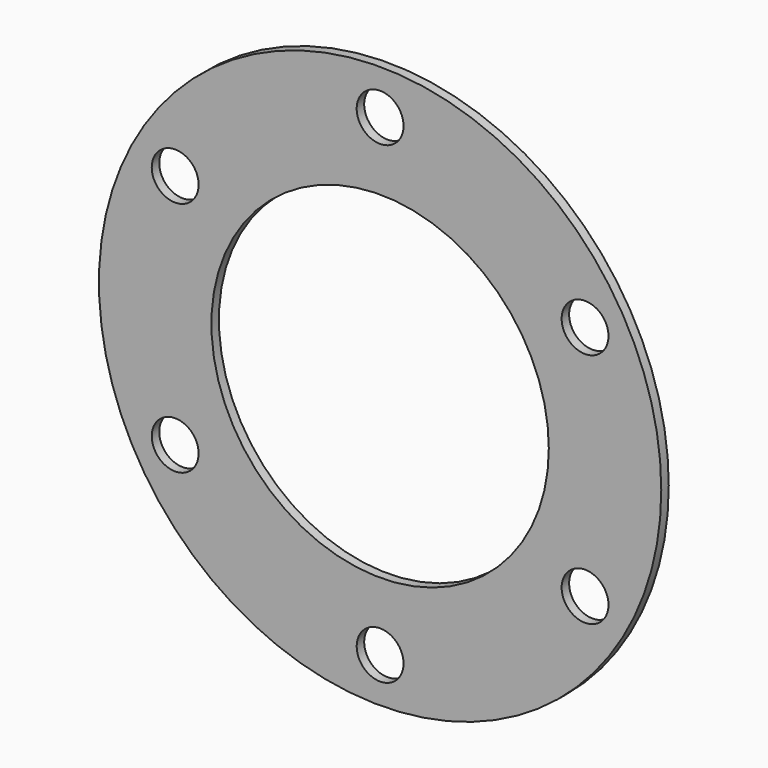
from build123d import *

# Parameters (mm, degrees)
F0_R            = 60
F0_R_2          = 36
F1_DEPTH        = 2
F2_R            = 5
F3_DEPTH        = 2.001
F3_COPIES_COUNT = 6


# Not quite as in the source:
# - a pattern or mirror of a feature is missing from the dataset's text; its kind, count and spacing are read off the source's solid


with BuildPart() as f1:
    # F0 (on Front) → F1 (new body)
    with BuildSketch(Plane.XZ):
        Circle(F0_R)
        Circle(F0_R_2, mode=Mode.SUBTRACT)
    extrude(amount=F1_DEPTH)

    # F2 (on face) → F3 (cut, through all)
    with BuildSketch(Plane.XZ.offset(2)):
        with Locations((0, 50.5)):
            Circle(F2_R)
    f3 = extrude(amount=-F3_DEPTH, mode=Mode.SUBTRACT)

    # F3_copies: F3 ×6 about axis
    f3_copies_axis = Axis((0, 0, 0), (0, 1, 0))
    for i in range(1, F3_COPIES_COUNT):
        add(f3.rotate(f3_copies_axis, i * 360 / F3_COPIES_COUNT), mode=Mode.SUBTRACT)


solid = f1.part
